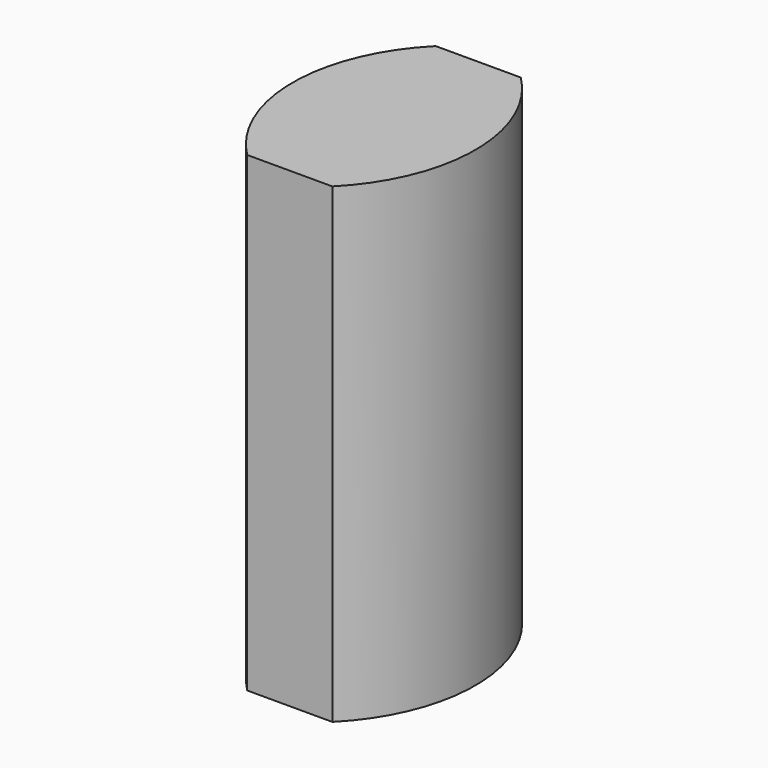
from build123d import *

# Parameters (mm, degrees)
F1_DEPTH               = 10
F2_DEPTH               = 15.1
DRAFT_F2_DRAFTED_ANGLE = -6
F3_R                   = 13
F4_DEPTH               = 3
F4_FACE_R              = 13
F5_DEPTH               = 72
F7_DEPTH               = 3


# Not quite as in the source:
# - an extrude with a draft is written as a straight extrude whose walls are then drafted


with BuildPart() as f1:
    # F0 (on Top) → F1 (new body)
    with BuildSketch(Plane.XY):
        with BuildLine():
            ThreePointArc((7.9466340877, -22.0000007098), (17.0456916094, 0), (7.9466340877, 22.0000007098))
            Line((7.9466340877, 22.0000007098), (-7.9466340877, 22.0000007098))
            ThreePointArc((-7.9466340877, 22.0000007098), (-17.0456916094, 0), (-7.9466340877, -22.0000007098))
            Line((-7.9466340877, -22.0000007098), (7.9466340877, -22.0000007098))
        make_face()
        with BuildLine():
            ThreePointArc((6.6648721695, 19), (14.0456908996, 0), (6.6648721695, -19))
            Line((6.6648721695, -19), (-6.6648721695, -19))
            ThreePointArc((-6.6648721695, -19), (-14.0456908996, 0), (-6.6648721695, 19))
            Line((-6.6648721695, 19), (6.6648721695, 19))
        make_face(mode=Mode.SUBTRACT)
    extrude(amount=-F1_DEPTH)


with BuildPart() as f2_drafted:
    # F0 (on Top) → F2 (new body)
    with BuildSketch(Plane.XY):
        with BuildLine():
            Line((-6.6648721695, -19), (6.6648721695, -19))
            ThreePointArc((6.6648721695, -19), (14.0456908996, 0), (6.6648721695, 19))
            Line((6.6648721695, 19), (-6.6648721695, 19))
            ThreePointArc((-6.6648721695, 19), (-14.0456908996, 0), (-6.6648721695, -19))
        make_face()
    extrude(amount=-F2_DEPTH)

    # draft_F2_drafted
    draft_f2_drafted_walls = [f2_drafted.faces().sort_by_distance(p)[0] for p in [
        (-14.0456908996, 0, -10.0666666667),
        (0, -19, -10.0666666667),
        (14.0456908996, 0, -10.0666666667),
        (0, 19, -10.0666666667),
    ]]
    draft(draft_f2_drafted_walls, neutral_plane=Plane(origin=(0, 0, 0), x_dir=(1, 0, 0), z_dir=(0, 0, -1)), angle=DRAFT_F2_DRAFTED_ANGLE)


with BuildPart() as f1_1:
    add(f1.part)

    # join_F2_drafted: cut F2_drafted
    add(f2_drafted.part, mode=Mode.SUBTRACT)

    # F3 (on face) + F1_face (on face) → F4 (join)
    with BuildSketch(Plane.XY):
        with BuildLine():
            ThreePointArc((-7.9466340877, 22.0000007098), (-17.0456916094, 0), (-7.9466340877, -22.0000007098))
            Line((-7.9466340877, -22.0000007098), (7.9466340877, -22.0000007098))
            ThreePointArc((7.9466340877, -22.0000007098), (17.0456916094, 0), (7.9466340877, 22.0000007098))
            Line((7.9466340877, 22.0000007098), (-7.9466340877, 22.0000007098))
        make_face()
        with BuildLine():
            ThreePointArc((11.9634722062, 10.6242803413), (14.9568638975, 5.6826246005), (16, 0))
            ThreePointArc((16, 0), (14.9568638975, -5.6826246005), (11.9634722062, -10.6242803413))
            ThreePointArc((11.9634722062, -10.6242803413), (9.685744243, -15.0472019666), (6.6648721695, -19))
            Line((6.6648721695, -19), (-6.6648721695, -19))
            ThreePointArc((-6.6648721695, -19), (-9.685744243, -15.0472019666), (-11.9634722062, -10.6242803413))
            ThreePointArc((-11.9634722062, -10.6242803413), (-16, 0), (-11.9634722062, 10.6242803413))
            ThreePointArc((-11.9634722062, 10.6242803413), (-9.685744243, 15.0472019666), (-6.6648721695, 19))
            Line((-6.6648721695, 19), (6.6648721695, 19))
            ThreePointArc((6.6648721695, 19), (9.685744243, 15.0472019666), (11.9634722062, 10.6242803413))
        make_face(mode=Mode.SUBTRACT)
        with BuildLine():
            ThreePointArc((-11.9634722062, 10.6242803413), (0, 16), (11.9634722062, 10.6242803413))
            ThreePointArc((11.9634722062, 10.6242803413), (9.685744243, 15.0472019666), (6.6648721695, 19))
            Line((6.6648721695, 19), (-6.6648721695, 19))
            ThreePointArc((-6.6648721695, 19), (-9.685744243, 15.0472019666), (-11.9634722062, 10.6242803413))
        make_face()
        with BuildLine():
            ThreePointArc((11.9634722062, -10.6242803413), (14.0456908996, 0), (11.9634722062, 10.6242803413))
            ThreePointArc((11.9634722062, 10.6242803413), (0, 16), (-11.9634722062, 10.6242803413))
            ThreePointArc((-11.9634722062, 10.6242803413), (-14.0456908996, 0), (-11.9634722062, -10.6242803413))
            ThreePointArc((-11.9634722062, -10.6242803413), (0, -16), (11.9634722062, -10.6242803413))
        make_face()
        Circle(F3_R, mode=Mode.SUBTRACT)
        with BuildLine():
            ThreePointArc((11.9634722062, -10.6242803413), (14.9568638975, -5.6826246005), (16, 0))
            ThreePointArc((16, 0), (14.9568638975, 5.6826246005), (11.9634722062, 10.6242803413))
            ThreePointArc((11.9634722062, 10.6242803413), (14.0456908996, 0), (11.9634722062, -10.6242803413))
        make_face()
        with BuildLine():
            ThreePointArc((6.6648721695, -19), (9.685744243, -15.0472019666), (11.9634722062, -10.6242803413))
            ThreePointArc((11.9634722062, -10.6242803413), (0, -16), (-11.9634722062, -10.6242803413))
            ThreePointArc((-11.9634722062, -10.6242803413), (-9.685744243, -15.0472019666), (-6.6648721695, -19))
            Line((-6.6648721695, -19), (6.6648721695, -19))
        make_face()
    with BuildSketch(Plane.XY):
        with BuildLine():
            Line((7.9466340877, 22.0000007098), (-7.9466340877, 22.0000007098))
            ThreePointArc((-7.9466340877, 22.0000007098), (-17.0456916094, 0), (-7.9466340877, -22.0000007098))
            Line((-7.9466340877, -22.0000007098), (7.9466340877, -22.0000007098))
            ThreePointArc((7.9466340877, -22.0000007098), (17.0456916094, 0), (7.9466340877, 22.0000007098))
        make_face()
        with BuildLine():
            ThreePointArc((6.6648721695, 19), (14.0456908996, 0), (6.6648721695, -19))
            Line((6.6648721695, -19), (-6.6648721695, -19))
            ThreePointArc((-6.6648721695, -19), (-14.0456908996, 0), (-6.6648721695, 19))
            Line((-6.6648721695, 19), (6.6648721695, 19))
        make_face(mode=Mode.SUBTRACT)
    extrude(amount=F4_DEPTH)

    # F3 (on face) + F4_face (on face) → F5 (join)
    with BuildSketch(Plane.XY):
        with BuildLine():
            ThreePointArc((-11.9634722062, -10.6242803413), (-14.0456908996, 0), (-11.9634722062, 10.6242803413))
            ThreePointArc((-11.9634722062, 10.6242803413), (-16, 0), (-11.9634722062, -10.6242803413))
        make_face()
        with BuildLine():
            ThreePointArc((11.9634722062, -10.6242803413), (14.0456908996, 0), (11.9634722062, 10.6242803413))
            ThreePointArc((11.9634722062, 10.6242803413), (0, 16), (-11.9634722062, 10.6242803413))
            ThreePointArc((-11.9634722062, 10.6242803413), (-14.0456908996, 0), (-11.9634722062, -10.6242803413))
            ThreePointArc((-11.9634722062, -10.6242803413), (0, -16), (11.9634722062, -10.6242803413))
        make_face()
        Circle(F3_R, mode=Mode.SUBTRACT)
        with BuildLine():
            ThreePointArc((11.9634722062, -10.6242803413), (14.9568638975, -5.6826246005), (16, 0))
            ThreePointArc((16, 0), (14.9568638975, 5.6826246005), (11.9634722062, 10.6242803413))
            ThreePointArc((11.9634722062, 10.6242803413), (14.0456908996, 0), (11.9634722062, -10.6242803413))
        make_face()
    with BuildSketch(Plane.XY.offset(3)):
        with BuildLine():
            ThreePointArc((-7.9466340877, 22.0000007098), (-17.0456916094, 0), (-7.9466340877, -22.0000007098))
            Line((-7.9466340877, -22.0000007098), (7.9466340877, -22.0000007098))
            ThreePointArc((7.9466340877, -22.0000007098), (17.0456916094, 0), (7.9466340877, 22.0000007098))
            Line((7.9466340877, 22.0000007098), (-7.9466340877, 22.0000007098))
        make_face()
        Circle(F4_FACE_R, mode=Mode.SUBTRACT)
    extrude(amount=F5_DEPTH)

    # F6 (on face) → F7 (join)
    with BuildSketch(Plane.XY.offset(75)):
        with BuildLine():
            ThreePointArc((-7.9466340877, 22.0000007098), (-17.0456916094, 0), (-7.9466340877, -22.0000007098))
            Line((-7.9466340877, -22.0000007098), (7.9466340877, -22.0000007098))
            ThreePointArc((7.9466340877, -22.0000007098), (17.0456916094, 0), (7.9466340877, 22.0000007098))
            Line((7.9466340877, 22.0000007098), (-7.9466340877, 22.0000007098))
        make_face()
    extrude(amount=F7_DEPTH)


solid = f1_1.part
